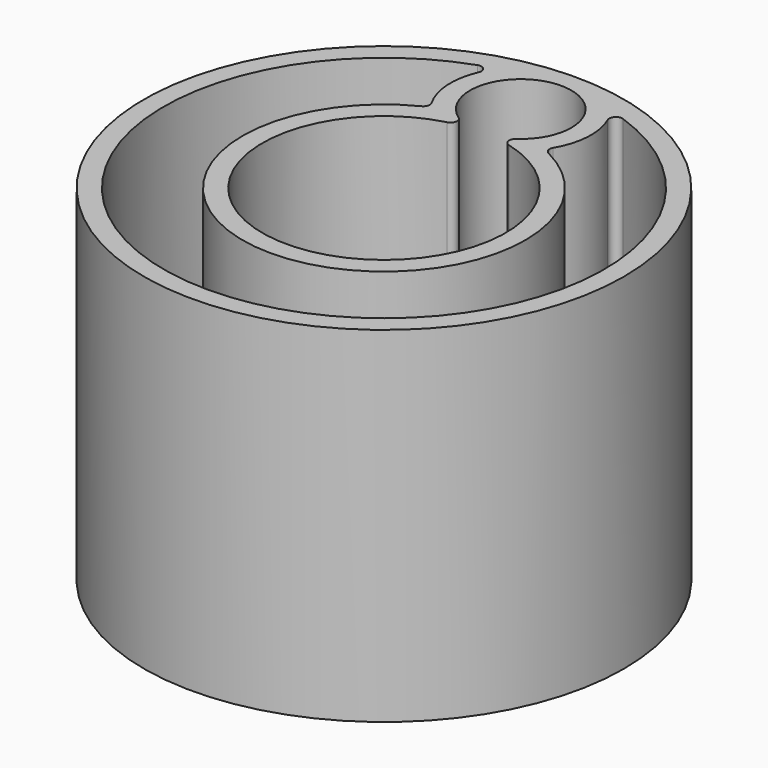
from build123d import *

# Parameters (mm, degrees)
F0_R     = 18.542
F0_R_2   = 3.175
F1_DEPTH = 7.62
F2_R     = 18.542
F3_DEPTH = 19.05
F4_R     = 0.508


with BuildPart() as f1:
    # F0 (on Top) → F1 (new body)
    with BuildSketch(Plane.XY):
        Circle(F0_R)
        with Locations((0, 13.208)):
            Circle(F0_R_2, mode=Mode.SUBTRACT)
    extrude(amount=F1_DEPTH)

    # F2 (on face) → F3 (join)
    with BuildSketch(Plane.XY.offset(7.62)):
        Circle(F2_R)
        with BuildLine():
            ThreePointArc((-4.3636460762, 16.44904), (-5.435558049, 13.2293554581), (-4.3889780516, 10.0013476923))
            ThreePointArc((-4.3889780516, 10.0013476923), (0, -10.922), (4.3889780516, 10.0013476923))
            ThreePointArc((4.3889780516, 10.0013476923), (5.435558049, 13.2293554581), (4.3636460762, 16.44904))
            ThreePointArc((4.3636460762, 16.44904), (0, -17.018), (-4.3636460762, 16.44904))
        make_face(mode=Mode.SUBTRACT)
        with BuildLine():
            ThreePointArc((-0.7465455676, 9.3683015385), (0, 17.1196), (0.7465455676, 9.3683015385))
            ThreePointArc((0.7465455676, 9.3683015385), (0, -9.398), (-0.7465455676, 9.3683015385))
        make_face(mode=Mode.SUBTRACT)
    extrude(amount=F3_DEPTH)

    # F4
    f4_edges = [f1.edges().sort_by_distance(p)[0] for p in [
        (0.746546, 9.368302, 17.145),
        (4.388978, 10.001348, 17.145),
        (4.363646, 16.44904, 17.145),
        (-4.388978, 10.001348, 17.145),
        (-4.363646, 16.44904, 17.145),
        (-0.746546, 9.368302, 17.145),
    ]]
    fillet(f4_edges, radius=F4_R)


solid = f1.part
